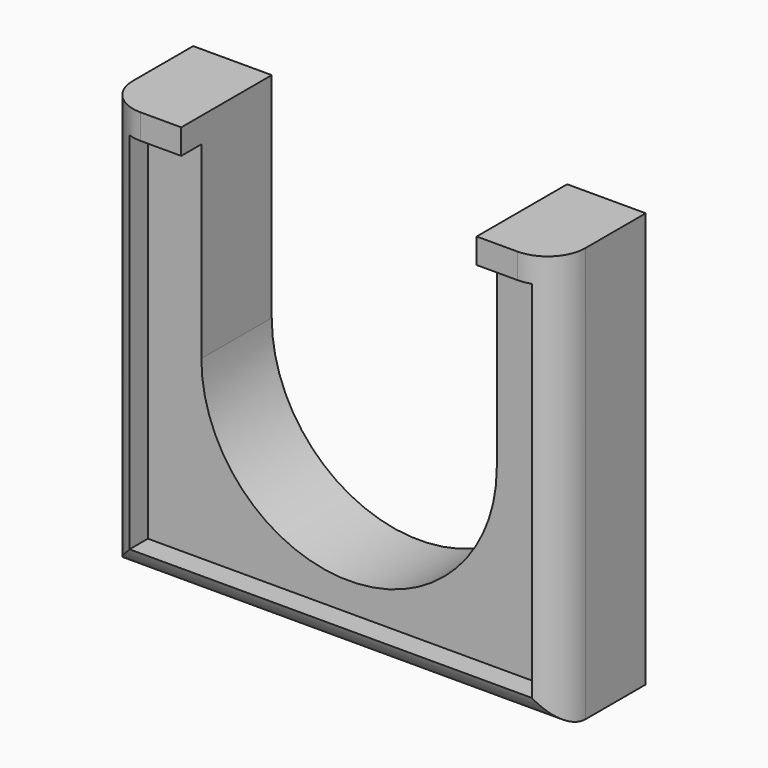
from build123d import *

# Parameters (mm, degrees)
F0_W        = 36
F0_H        = 33
F1_DEPTH    = 9
F3_DEPTH    = 25
F4_W        = 32
F4_H        = 29
F5_DEPTH    = 2
F6_R        = 0.75
F7_DEPTH    = 4
F8_T1_DEPTH = 48
F8_T3_DEPTH = 51


# Not quite as in the source:
# - a fillet or chamfer that OpenCascade refuses, or shapes differently, is made with other operations: its cross-section is extruded or revolved along the edge and cut away or added


with BuildPart() as f1:
    # F0 (on Front) → F1 (new body)
    with BuildSketch(Plane.XZ):
        with Locations((18, 16.5)):
            Rectangle(F0_W, F0_H)
    extrude(amount=F1_DEPTH)

    # F2 (on face) → F3 (cut)
    with BuildSketch(Plane.XZ.offset(9)):
        with BuildLine():
            ThreePointArc((6.25, 16), (18, 4.25), (29.75, 16))
            ThreePointArc((29.75, 16), (18, 27.75), (6.25, 16))
        make_face()
        with BuildLine():
            ThreePointArc((6.25, 16), (18, 27.75), (29.75, 16))
            Line((29.75, 16), (29.75, 33))
            Line((29.75, 33), (6.25, 33))
            Line((6.25, 33), (6.25, 16))
        make_face()
    extrude(amount=-F3_DEPTH, mode=Mode.SUBTRACT)

    # F4 (on face) → F5 (cut)
    with BuildSketch(Plane.XZ.offset(9)):
        with Locations((18, 16.5)):
            Rectangle(F4_W, F4_H)
    extrude(amount=-F5_DEPTH, mode=Mode.SUBTRACT)

    # F6 (on face) → F7 (cut)
    with BuildSketch(Plane(origin=(0, 0, 0), x_dir=(-1, 0, 0), z_dir=(0, 1, 0))):
        with Locations((-31.5, 30)):
            Circle(F6_R)
        with Locations((-3, 30)):
            Circle(F6_R)
        with Locations((-3, 3)):
            Circle(F6_R)
        with Locations((-31, 3)):
            Circle(F6_R)
    extrude(amount=-F7_DEPTH, mode=Mode.SUBTRACT)

    # F8: fillet of radius 3 on 3 edges, made by hand

    # F8_s2 → F8_t1 (cut)
    with BuildSketch(Plane.XY.offset(-7.5)):
        with BuildLine():
            ThreePointArc((33, -9), (35.1213203436, -8.1213203436), (36, -6))
            Line((36, -6), (36, -9))
            Line((36, -9), (33, -9))
        make_face()
        with BuildLine():
            ThreePointArc((0, -6), (0.8786796564, -8.1213203436), (3, -9))
            Line((3, -9), (0, -9))
            Line((0, -9), (0, -6))
        make_face()
    extrude(amount=F8_T1_DEPTH, mode=Mode.SUBTRACT)

    # F8_s4 → F8_t3 (cut)
    with BuildSketch(Plane.YZ.offset(-7.5)):
        with BuildLine():
            ThreePointArc((-6, 0), (-8.1213203436, 0.8786796564), (-9, 3))
            Line((-9, 3), (-9, 0))
            Line((-9, 0), (-6, 0))
        make_face()
    extrude(amount=F8_T3_DEPTH, mode=Mode.SUBTRACT)


solid = f1.part
